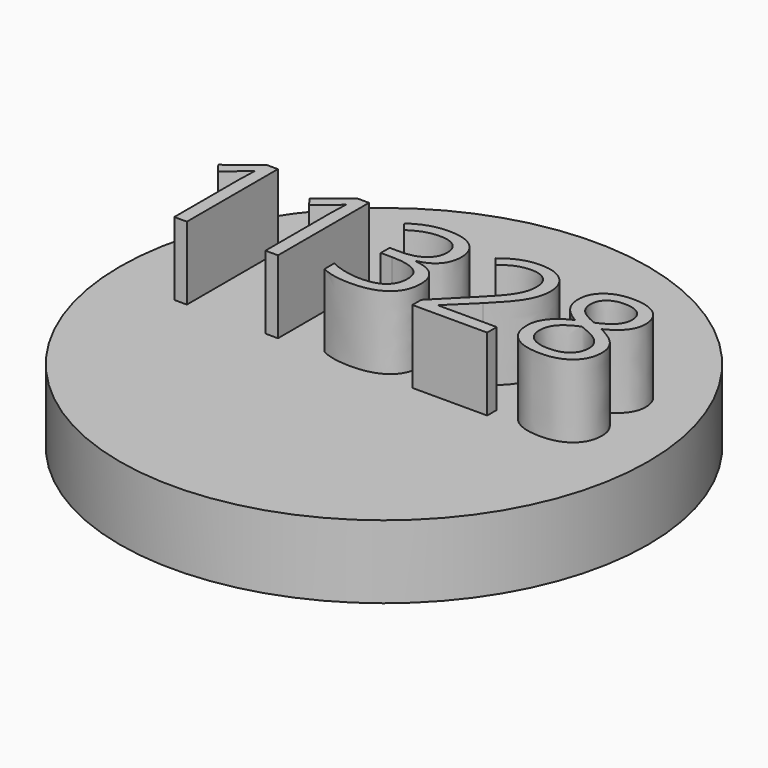
from build123d import *

# Parameters (mm, degrees)
F0_R         = 91.8519390569
F1_DEPTH     = 25.4
F2_TEXT_SIZE = 55.423223724
F3_DEPTH     = 25.4


# Not quite as in the source:
# - Text() gives the source's letters only with a copy of the font that has no kerning and outlines rounded to 1/6400 em; it was checked with that copy


with BuildPart() as f1:
    # F0 (on Top) → F1 (new body)
    with BuildSketch(Plane.XY):
        Circle(F0_R)
    extrude(amount=F1_DEPTH)

    # F2 (on face) → F3 (join)
    with BuildSketch(Plane.XY.offset(25.4)):
        with Locations((-83.0119363964, -6.108882837)):
            Text('11328', F2_TEXT_SIZE, font='Open Sans', text_align=(TextAlign.LEFT, TextAlign.BOTTOM))
    extrude(amount=F3_DEPTH)


solid = f1.part
